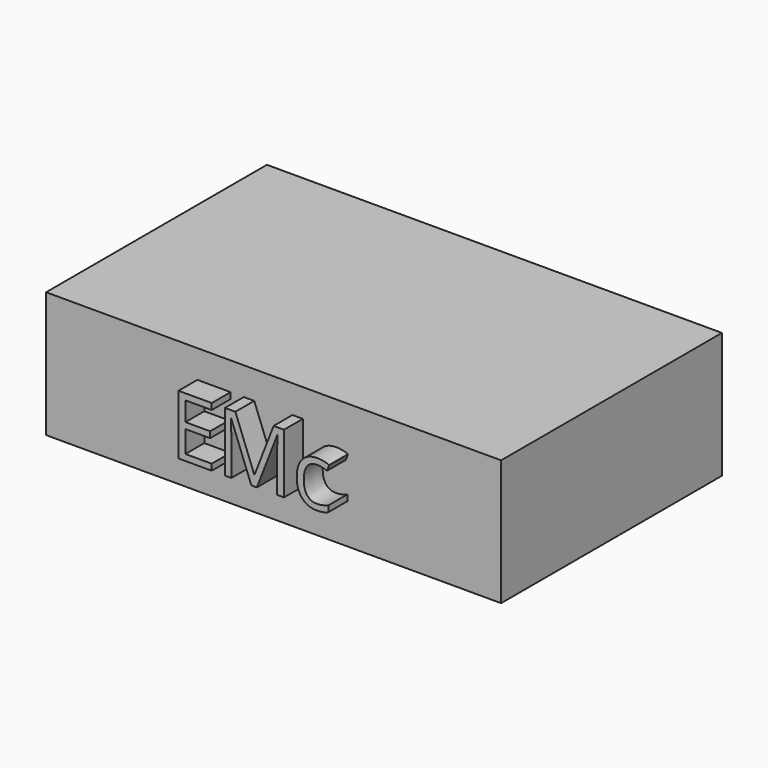
from build123d import *

# Parameters (mm, degrees)
F0_W         = 482.4
F0_H         = 133.35
F1_DEPTH     = 292.6
F2_TEXT_SIZE = 88.5186535824
F3_DEPTH     = 25


# Not quite as in the source:
# - Text() gives the source's letters only with a copy of the font that has no kerning and outlines rounded to 1/6400 em; it was checked with that copy


with BuildPart() as f1:
    # F0 (on Front) → F1 (new body)
    with BuildSketch(Plane.XZ):
        Rectangle(F0_W, F0_H)
    extrude(amount=F1_DEPTH)

    # F2 (on face) → F3 (join)
    with BuildSketch(Plane.XZ.offset(292.6)):
        with Locations((-89.5107388496, -26.1476505548)):
            Text('EMc', F2_TEXT_SIZE, font='Open Sans', text_align=(TextAlign.LEFT, TextAlign.BOTTOM))
    extrude(amount=F3_DEPTH)


solid = f1.part
